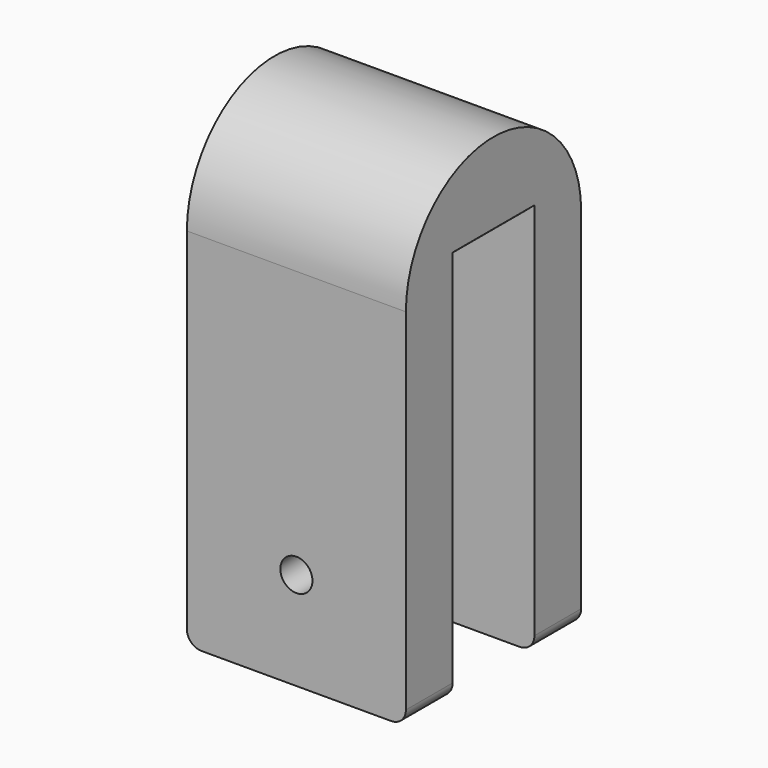
from build123d import *

# Parameters (mm, degrees)
F1_DEPTH     = 15
F3_DEPTH     = 3.5
F4_R         = 1.1
F5_DEPTH     = 15.001
F6_R         = 1
F7_TEXT_SIZE = 13.8888888889
F8_DEPTH     = 1
F9_R         = 1.6
F9_R_2       = 1.1
F10_DEPTH    = 5


# Not quite as in the source:
# - Text() gives the source's letters only with a copy of the font that has no kerning and outlines rounded to 1/6400 em; it was checked with that copy


with BuildPart() as f1:
    # F0 (on Right) → F1 (new body)
    with BuildSketch(Plane.YZ):
        with BuildLine():
            Line((7.5, -25), (7.5, 0))
            ThreePointArc((7.5, 0), (0, 7.5), (-7.5, 0))
            Line((-7.5, 0), (-7.5, -25))
            Line((-7.5, -25), (7.5, -25))
        make_face()
    extrude(amount=F1_DEPTH)

    # F2 (on Front) → F3 (cut, symmetric)
    with BuildSketch(Plane.XZ):
        with BuildLine():
            Line((-0.4070811511, -31.5200583303), (15.4324545424, -31.5200583303))
            Line((15.4324545424, -31.5200583303), (15.4324545424, 2.3792280619))
            ThreePointArc((15.4324545424, 2.3792280619), (7.518280675, -0.9999848098), (-0.4070811511, 2.3529046253))
            Line((-0.4070811511, 2.3529046253), (-0.4070811511, -31.5200583303))
        make_face()
    extrude(amount=F3_DEPTH, both=True, mode=Mode.SUBTRACT)

    # F4 (on face) → F5 (cut, through all)
    with BuildSketch(Plane(origin=(0, 7.5, 0), x_dir=(-1, 0, 0), z_dir=(0, 1, 0))):
        with Locations((-7.5, -18.2978641242)):
            Circle(F4_R)
    extrude(amount=-F5_DEPTH, mode=Mode.SUBTRACT)

    # F6
    f6_edges = [f1.edges().sort_by_distance(p)[0] for p in [
        (15, 5.5, -25),
        (15, -5.5, -25),
        (0, 5.5, -25),
        (0, -5.5, -25),
    ]]
    fillet(f6_edges, radius=F6_R)

    # F7 (on face) → F8 (cut)
    with BuildSketch(Plane(origin=(0, 7.5, 0), x_dir=(-1, 0, 0), z_dir=(0, 1, 0))):
        with Locations((-12.4197048611, -12.5)):
            Text('C', F7_TEXT_SIZE, font='Tinos', font_style=FontStyle.BOLD, text_align=(TextAlign.LEFT, TextAlign.BOTTOM))
    extrude(amount=-F8_DEPTH, mode=Mode.SUBTRACT)

    # F9 (on face) → F10 (cut)
    with BuildSketch(Plane(origin=(0, 7.5, 0), x_dir=(-1, 0, 0), z_dir=(0, 1, 0))):
        with Locations((-7.5, -18.2978641242)):
            Circle(F9_R)
        with Locations((-7.5, -18.2978641242)):
            Circle(F9_R_2, mode=Mode.SUBTRACT)
    extrude(amount=-F10_DEPTH, mode=Mode.SUBTRACT)


solid = f1.part
